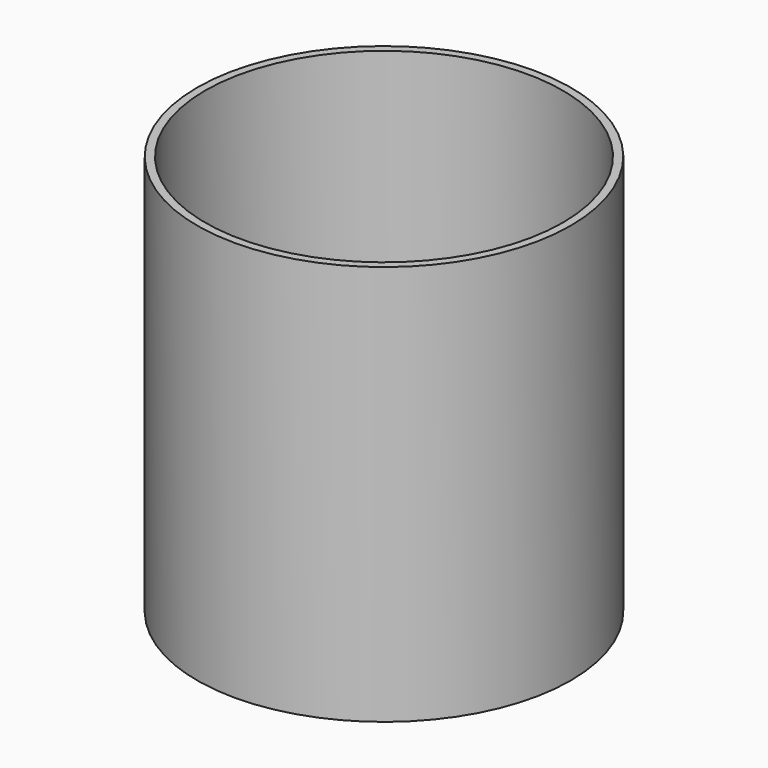
from build123d import *

# Parameters (mm, degrees)
F0_R         = 35
F1_DEPTH     = 75
F2_R         = 33.5
F3_DEPTH     = 70
F4_TEXT_SIZE = 6.1913514559
F5_DEPTH     = 5.001


# Not quite as in the source:
# - Text() gives the source's letters only with a copy of the font that has no kerning and outlines rounded to 1/6400 em; it was checked with that copy


with BuildPart() as f1:
    # F0 (on Top) → F1 (new body)
    with BuildSketch(Plane.XY):
        Circle(F0_R)
    extrude(amount=F1_DEPTH)

    # F2 (on face) → F3 (cut)
    with BuildSketch(Plane.XY.offset(75)):
        Circle(F2_R)
    extrude(amount=-F3_DEPTH, mode=Mode.SUBTRACT)

    # F4 (on face) → F5 (cut, through all)
    with BuildSketch(Plane.XY.offset(5)):
        with Locations((-13.1988143722, 10.2983738504)):
            Text('Prof Stols', F4_TEXT_SIZE, font='Open Sans', text_align=(TextAlign.LEFT, TextAlign.BOTTOM))
        with Locations((-24.4603022313, 1.8781358704)):
            Text('Keeping together', F4_TEXT_SIZE, font='Open Sans', text_align=(TextAlign.LEFT, TextAlign.BOTTOM))
        with Locations((-3.5461104929, -6.5421021097)):
            Text('the', F4_TEXT_SIZE, font='Open Sans', text_align=(TextAlign.LEFT, TextAlign.BOTTOM))
        with Locations((-14.8075983521, -14.9623400898)):
            Text('Coasters', F4_TEXT_SIZE, font='Open Sans', text_align=(TextAlign.LEFT, TextAlign.BOTTOM))
    extrude(amount=-F5_DEPTH, mode=Mode.SUBTRACT)


solid = f1.part
